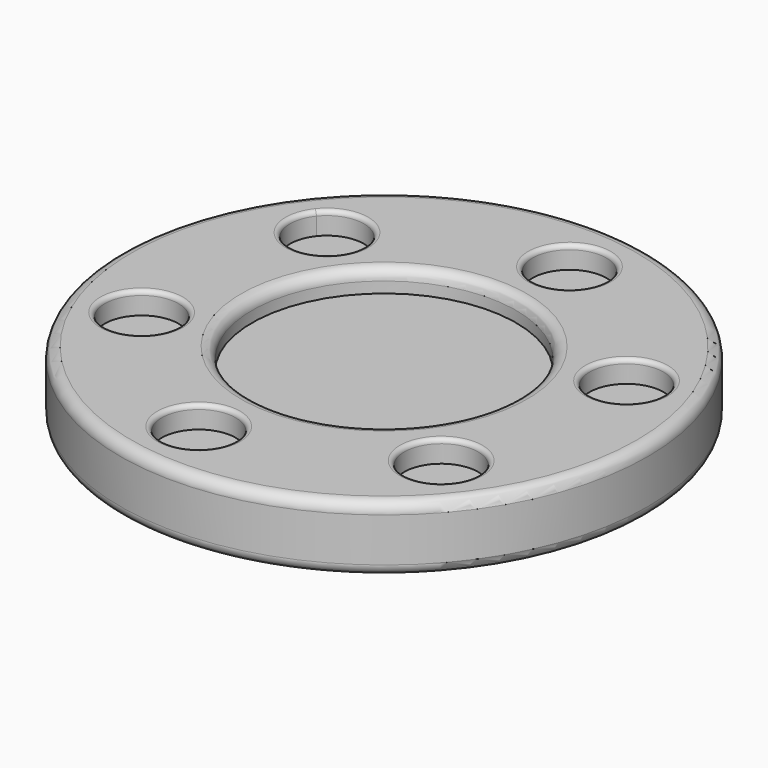
from build123d import *

# Parameters (mm, degrees)
F1_DEPTH = 50.8
F0_R     = 42.6318264633
F2_DEPTH = 76.2
F3_R     = 12.7
F4_R     = 5.08


with BuildPart() as f1:
    # F0 (on Top) → F1 (new body)
    with BuildSketch(Plane.XY):
        with BuildLine():
            ThreePointArc((152.4, 0), (50.0231829172, 143.9563863496), (-119.5611702209, 94.5033680638))
            ThreePointArc((-119.5611702209, 94.5033680638), (-50.0231829172, -143.9563863496), (152.4, 0))
        make_face()
    extrude(amount=F1_DEPTH)

    # F0 (on Top) → F2 (join)
    with BuildSketch(Plane.XY):
        with BuildLine():
            ThreePointArc((-239.1223404418, 189.0067361277), (-100.0463658344, -287.9127726992), (304.8, 0))
            ThreePointArc((304.8, 0), (100.0463658344, 287.9127726992), (-239.1223404418, 189.0067361277))
        make_face()
        with Locations((-33.092598564, -226.1920421241)):
            Circle(F0_R, mode=Mode.SUBTRACT)
        with Locations((-212.4343538954, -84.4369900284)):
            Circle(F0_R, mode=Mode.SUBTRACT)
        with Locations((179.3417553314, -141.7550520957)):
            Circle(F0_R, mode=Mode.SUBTRACT)
        with BuildLine():
            ThreePointArc((-145.8961446974, 115.3190206817), (-205.7777867454, 108.3094414618), (-212.7873659653, 168.1910835098))
            ThreePointArc((-212.7873659653, 168.1910835098), (-165.3484505199, 182.0248925232), (-136.709928868, 141.7550520957))
            ThreePointArc((-136.709928868, 141.7550520957), (-139.0719149039, 127.7617472843), (-145.8961446974, 115.3190206817))
        make_face(mode=Mode.SUBTRACT)
        with BuildLine():
            ThreePointArc((152.4, 0), (-50.0231829172, -143.9563863496), (-119.5611702209, 94.5033680638))
            ThreePointArc((-119.5611702209, 94.5033680638), (50.0231829172, 143.9563863496), (152.4, 0))
        make_face(mode=Mode.SUBTRACT)
        with Locations((212.4343538954, 84.4369900284)):
            Circle(F0_R, mode=Mode.SUBTRACT)
        with Locations((33.092598564, 226.1920421241)):
            Circle(F0_R, mode=Mode.SUBTRACT)
    extrude(amount=F2_DEPTH)

    # F3
    f3_edges = [f1.edges().sort_by_distance(p)[0] for p in [
        (-304.8, 0, 76.2),
        (-304.8, 0, 0),
        (-75.724425, -226.192042, 0),
        (-255.06618, -84.43699, 0),
        (136.709929, -141.755052, 0),
        (-221.973582, 141.755052, 0),
        (169.802527, 84.43699, 0),
        (-9.539228, 226.192042, 0),
        (119.56117, -94.503368, 76.2),
    ]]
    fillet(f3_edges, radius=F3_R)

    # F4
    f4_edges = [f1.edges().sort_by_distance(p)[0] for p in [
        (-255.06618, -84.43699, 76.2),
        (-221.973582, 141.755052, 76.2),
        (-9.539228, 226.192042, 76.2),
        (169.802527, 84.43699, 76.2),
        (-75.724425, -226.192042, 76.2),
        (136.709929, -141.755052, 76.2),
    ]]
    fillet(f4_edges, radius=F4_R)


with BuildPart() as f1b:
    # F0 (on Top) → F1, piece 2 (new body)
    with BuildSketch(Plane.XY):
        with Locations((-33.092598564, -226.1920421241)):
            Circle(F0_R)
    extrude(amount=F1_DEPTH)


with BuildPart() as f1c:
    # F0 (on Top) → F1, piece 3 (new body)
    with BuildSketch(Plane.XY):
        with Locations((179.3417553314, -141.7550520957)):
            Circle(F0_R)
    extrude(amount=F1_DEPTH)


with BuildPart() as f1d:
    # F0 (on Top) → F1, piece 4 (new body)
    with BuildSketch(Plane.XY):
        with Locations((212.4343538954, 84.4369900284)):
            Circle(F0_R)
    extrude(amount=F1_DEPTH)


with BuildPart() as f1e:
    # F0 (on Top) → F1, piece 5 (new body)
    with BuildSketch(Plane.XY):
        with Locations((33.092598564, 226.1920421241)):
            Circle(F0_R)
    extrude(amount=F1_DEPTH)


with BuildPart() as f1f:
    # F0 (on Top) → F1, piece 6 (new body)
    with BuildSketch(Plane.XY):
        with BuildLine():
            ThreePointArc((-136.709928868, 141.7550520957), (-165.3484505199, 182.0248925232), (-212.7873659653, 168.1910835098))
            Line((-212.7873659653, 168.1910835098), (-145.8961446974, 115.3190206817))
            ThreePointArc((-145.8961446974, 115.3190206817), (-139.0719149039, 127.7617472843), (-136.709928868, 141.7550520957))
        make_face()
        with BuildLine():
            Line((-145.8961446974, 115.3190206817), (-212.7873659653, 168.1910835098))
            ThreePointArc((-212.7873659653, 168.1910835098), (-205.7777867454, 108.3094414618), (-145.8961446974, 115.3190206817))
        make_face()
    extrude(amount=F1_DEPTH)


with BuildPart() as f1g:
    # F0 (on Top) → F1, piece 7 (new body)
    with BuildSketch(Plane.XY):
        with Locations((-212.4343538954, -84.4369900284)):
            Circle(F0_R)
    extrude(amount=F1_DEPTH)


solid = Compound([f1.part, f1b.part, f1c.part, f1d.part, f1e.part, f1f.part, f1g.part])
